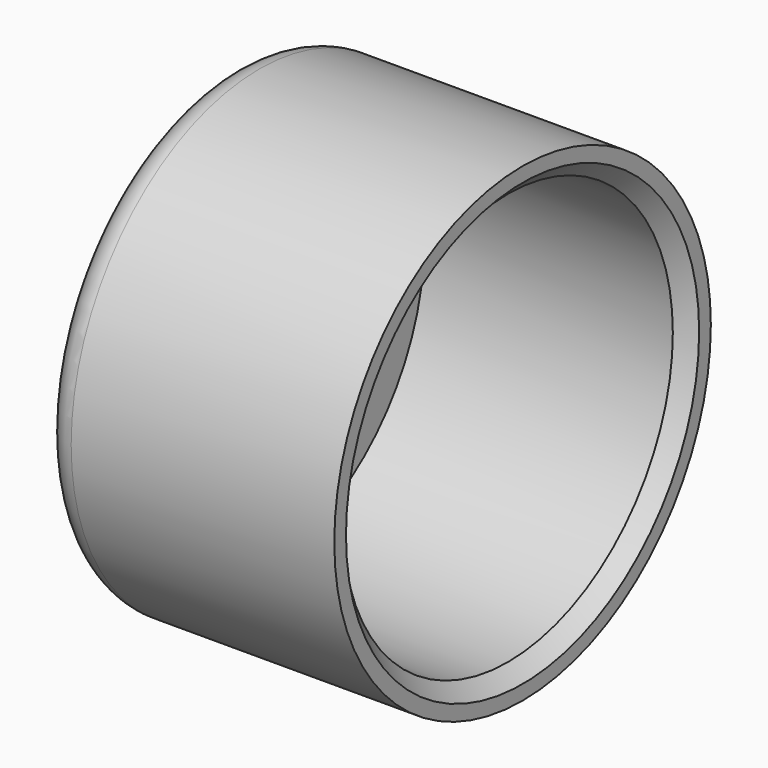
from build123d import *

# Parameters (mm, degrees)
F0_R         = 16.1
F0_R_2       = 14.1
F1_DEPTH     = 20
F2_DEPTH     = 2
F3_SIZE      = 1
F4_R         = 2
F5_TEXT_SIZE = 14.4986060655
F6_DEPTH     = 1


# Not quite as in the source:
# - Text() gives the source's letters only with a copy of the font that has no kerning and outlines rounded to 1/6400 em; it was checked with that copy


with BuildPart() as f1:
    # F0 (on Right) → F1 (new body)
    with BuildSketch(Plane.YZ):
        Circle(F0_R)
        Circle(F0_R_2, mode=Mode.SUBTRACT)
    extrude(amount=F1_DEPTH)

    # F0 (on Right) → F2 (join)
    with BuildSketch(Plane.YZ):
        Circle(F0_R_2)
    extrude(amount=F2_DEPTH)

    # F3
    f3_edges = [f1.edges().sort_by_distance(p)[0] for p in [
        (20, -14.1, 0),
    ]]
    chamfer(f3_edges, length=F3_SIZE)

    # F4
    f4_edges = [f1.edges().sort_by_distance(p)[0] for p in [
        (0, -16.1, 0),
    ]]
    fillet(f4_edges, radius=F4_R)

    # F5 (on face) → F6 (cut)
    with BuildSketch(Plane(origin=(0, 0, 0), x_dir=(0, -1, 0), z_dir=(-1, 0, 0))):
        with Locations((-4.7828181414, -5.363588687)):
            Text('P', F5_TEXT_SIZE, font='Open Sans', font_style=FontStyle.BOLD, text_align=(TextAlign.LEFT, TextAlign.BOTTOM))
    extrude(amount=-F6_DEPTH, mode=Mode.SUBTRACT)


solid = f1.part
